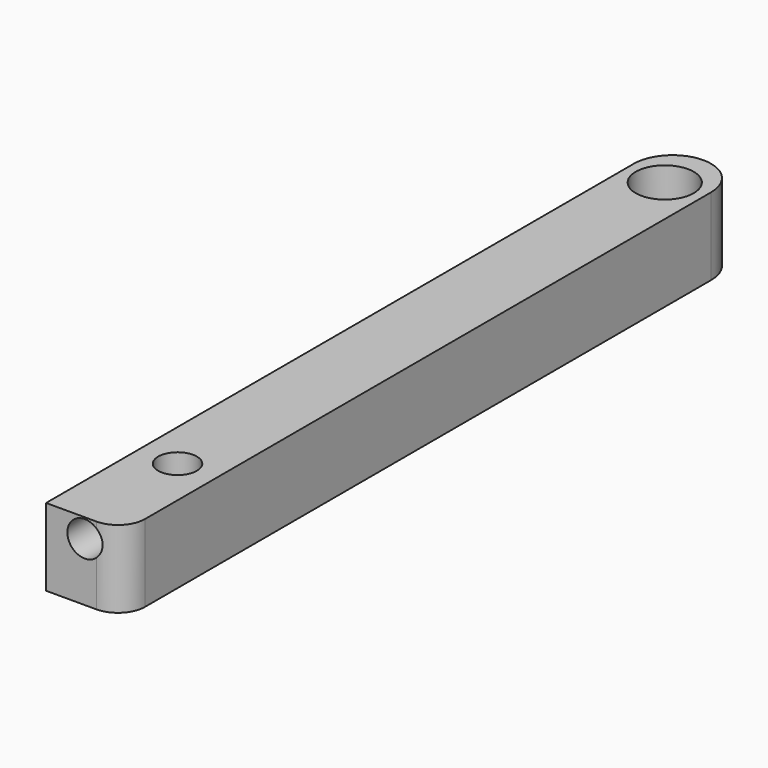
from build123d import *

# Parameters (mm, degrees)
F0_W        = 25.4
F0_H        = 254
F0_R        = 9.525
F1_DEPTH    = 25.4
F2_R        = 12.69999
F3_R        = 5.715
F4_DEPTH    = 26.67
F6_DEPTH    = 25.4
F7_T1_DEPTH = 69.85


# Not quite as in the source:
# - a fillet or chamfer that OpenCascade refuses, or shapes differently, is made with other operations: its cross-section is extruded or revolved along the edge and cut away or added
# - a fillet or chamfer is up to 0.001 mm smaller than in the source, because OpenCascade refuses the exact size


with BuildPart() as f1:
    # F0 (on Top) → F1 (new body)
    with BuildSketch(Plane.XY):
        with Locations((-33.2050182253, 13.4569510469)):
            Rectangle(F0_W, F0_H)
        with Locations((-33.2050182253, 124.5819510469)):
            Circle(F0_R, mode=Mode.SUBTRACT)
    extrude(amount=-F1_DEPTH)

    # F2 (radius 12.7 in the source; OpenCascade refuses exactly that, so slightly less here)
    f2_edges = [f1.edges().sort_by_distance(p)[0] for p in [
        (-45.905018, 140.456951, -12.7),
        (-20.505018, 140.456951, -12.7),
    ]]
    fillet(f2_edges, radius=F2_R)

    # F3 (on face) → F4 (cut)
    with BuildSketch(Plane.XZ.offset(113.5430489531)):
        with Locations((-33.2050182253, -6.2401448376)):
            Circle(F3_R)
    extrude(amount=-F4_DEPTH, mode=Mode.SUBTRACT)

    # F5 (on face) → F6 (cut)
    with BuildSketch(Plane(origin=(0, 0, -25.4), x_dir=(1, 0, 0), z_dir=(0, 0, -1))):
        with BuildLine():
            ThreePointArc((-33.2050182253, 81.7930489531), (-37.6951462858, 70.9529208925), (-26.8550182253, 75.4430489531))
            ThreePointArc((-26.8550182253, 75.4430489531), (-28.7148901648, 79.9331770136), (-33.2050182253, 81.7930489531))
        make_face()
    extrude(amount=-F6_DEPTH, mode=Mode.SUBTRACT)

    # F7: fillet of radius 8.89 on 1 edges, made by hand

    # F7_s2 → F7_t1 (cut)
    with BuildSketch(Plane.XY.offset(-47.625)):
        with BuildLine():
            ThreePointArc((-20.5050182253, -104.6530489531), (-23.1088389406, -110.9392282378), (-29.3950182253, -113.5430489531))
            Line((-29.3950182253, -113.5430489531), (-20.5050182253, -113.5430489531))
            Line((-20.5050182253, -113.5430489531), (-20.5050182253, -104.6530489531))
        make_face()
    extrude(amount=F7_T1_DEPTH, mode=Mode.SUBTRACT)


solid = f1.part
